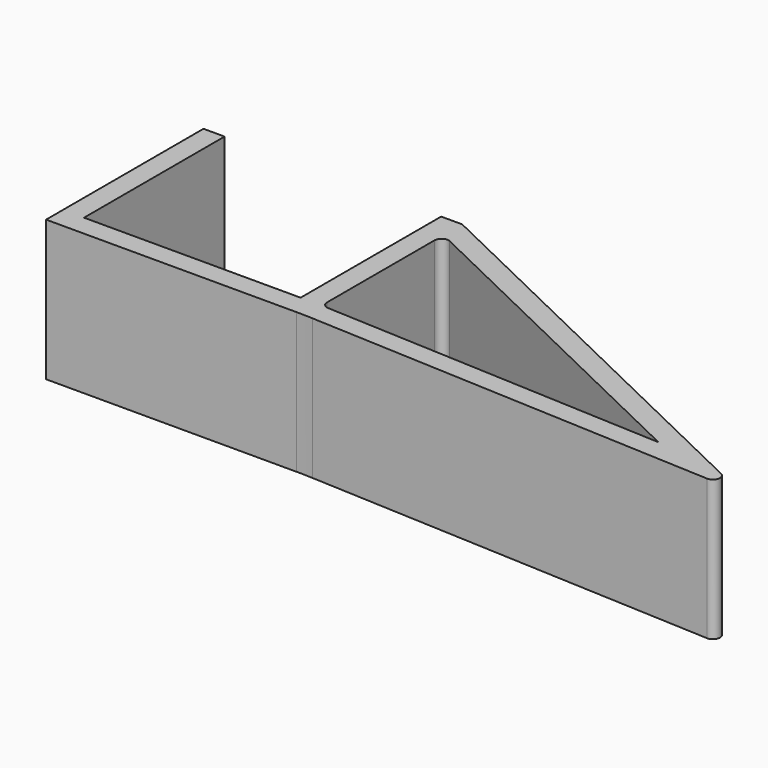
from build123d import *

# Parameters (mm, degrees)
F2_DEPTH = 20


with BuildPart() as f2:
    # F1 (on Top) → F2 (new body)
    with BuildSketch(Plane.XY):
        with BuildLine():
            Line((-36.82, 0), (-1.1677719632, 0))
            ThreePointArc((-1.1677719632, 0), (-0.0003183659, -0.0136313372), (1.1664986733, -0.0545179161))
            Line((1.1664986733, -0.0545179161), (59.4533145873, -2.7786322345))
            ThreePointArc((59.4533145873, -2.7786322345), (60.4694396966, -2.0250523194), (59.9340803732, -0.8788484453))
            Line((59.9340803732, -0.8788484453), (0, 28))
            Line((0, 28), (-3, 28))
            Line((-3, 28), (-3, 3))
            Line((-3, 3), (-33.82, 3))
            Line((-33.82, 3), (-33.82, 28))
            Line((-33.82, 28), (-36.82, 28))
            Line((-36.82, 28), (-36.82, 0))
        make_face()
        with BuildLine():
            ThreePointArc((0.9533145873, 2.9587201802), (0.2765757079, 3.267226104), (0, 3.9576298219))
            Line((0, 3.9576298219), (0, 23.0780246214))
            ThreePointArc((0, 23.0780246214), (0.4680603292, 23.924806876), (1.4340803732, 23.9788987689))
            Line((1.4340803732, 23.9788987689), (49.7960707162, 0.6759869543))
            Line((49.7960707162, 0.6759869543), (0.9533145873, 2.9587201802))
        make_face(mode=Mode.SUBTRACT)
    extrude(amount=F2_DEPTH)


solid = f2.part
